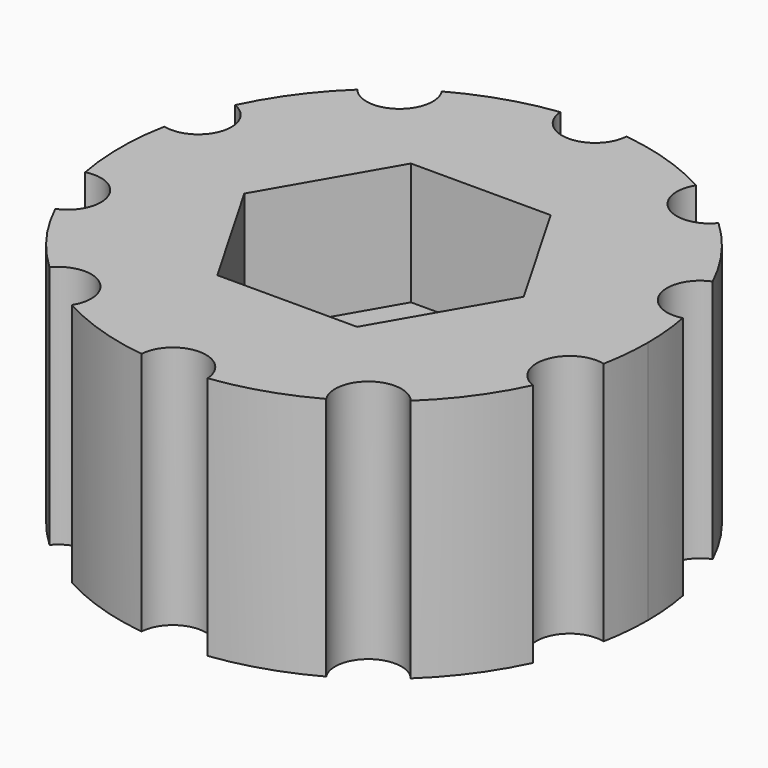
from build123d import *

# Parameters (mm, degrees)
F1_DEPTH = 10
F2_R     = 3
F3_DEPTH = 10.001
F4_R     = 3
F5_DEPTH = 5


with BuildPart() as f1:
    # F0 (on Top) → F1 (new body)
    with BuildSketch(Plane.XY):
        with BuildLine():
            ThreePointArc((10.6036903919, -2.023307953), (10.747066176, -1.0161661329), (10.795, 0))
            ThreePointArc((10.795, 0), (10.747066176, 1.0161661329), (10.6036903919, 2.023307953))
            ThreePointArc((10.6036903919, 2.023307953), (8.9778667931, 2.9170857512), (9.7678363058, 4.5958023134))
            ThreePointArc((9.7678363058, 4.5958023134), (8.7333384543, 6.3451417985), (7.3892951545, 7.8695833511))
            ThreePointArc((7.3892951545, 7.8695833511), (5.5486268246, 7.6370296448), (5.2010007473, 9.4594723017))
            ThreePointArc((5.2010007473, 9.4594723017), (3.3358384543, 10.2666550934), (1.352440321, 10.7099453863))
            ThreePointArc((1.352440321, 10.7099453863), (0, 9.4398877872), (-1.352440321, 10.7099453863))
            ThreePointArc((-1.352440321, 10.7099453863), (-3.3358384543, 10.2666550934), (-5.2010007473, 9.4594723017))
            ThreePointArc((-5.2010007473, 9.4594723017), (-5.0438407916, 9.1114188675), (-4.9900295857, 8.7333384543))
            ThreePointArc((-4.9900295857, 8.7333384543), (-5.8861297374, 7.4583337339), (-7.3892951545, 7.8695833511))
            ThreePointArc((-7.3892951545, 7.8695833511), (-8.7333384543, 6.3451417985), (-9.7678363058, 4.5958023134))
            ThreePointArc((-9.7678363058, 4.5958023134), (-9.1458775641, 4.0975384208), (-8.9115428806, 3.3358384543))
            ThreePointArc((-8.9115428806, 3.3358384543), (-9.4361105551, 2.2650794341), (-10.6036903919, 2.023307953))
            ThreePointArc((-10.6036903919, 2.023307953), (-10.795, 0), (-10.6036903919, -2.023307953))
            ThreePointArc((-10.6036903919, -2.023307953), (-9.4361105551, -2.2650794341), (-8.9115428806, -3.3358384543))
            ThreePointArc((-8.9115428806, -3.3358384543), (-9.1458775641, -4.0975384208), (-9.7678363058, -4.5958023134))
            ThreePointArc((-9.7678363058, -4.5958023134), (-8.7333384543, -6.3451417985), (-7.3892951545, -7.8695833511))
            ThreePointArc((-7.3892951545, -7.8695833511), (-5.8861297374, -7.4583337339), (-4.9900295857, -8.7333384543))
            ThreePointArc((-4.9900295857, -8.7333384543), (-5.0438407916, -9.1114188675), (-5.2010007473, -9.4594723017))
            ThreePointArc((-5.2010007473, -9.4594723017), (-3.3358384543, -10.2666550934), (-1.352440321, -10.7099453863))
            ThreePointArc((-1.352440321, -10.7099453863), (0, -9.4398877872), (1.352440321, -10.7099453863))
            ThreePointArc((1.352440321, -10.7099453863), (3.3358384543, -10.2666550934), (5.2010007473, -9.4594723017))
            ThreePointArc((5.2010007473, -9.4594723017), (5.5486268246, -7.6370296448), (7.3892951545, -7.8695833511))
            ThreePointArc((7.3892951545, -7.8695833511), (8.7333384543, -6.3451417985), (9.7678363058, -4.5958023134))
            ThreePointArc((9.7678363058, -4.5958023134), (8.9778667931, -2.9170857512), (10.6036903919, -2.023307953))
        make_face()
    extrude(amount=F1_DEPTH)

    # F2 (on face) → F3 (cut, through all)
    with BuildSketch(Plane.XY.offset(10)):
        Circle(F2_R)
    extrude(amount=-F3_DEPTH, mode=Mode.SUBTRACT)

    # F4 (on face) → F5 (cut)
    with BuildSketch(Plane.XY.offset(10)):
        Polygon((2.8578838325, -4.95), (5.715767665, 0), (2.8578838325, 4.95), (-2.8578838325, 4.95), (-5.715767665, 0), (-2.8578838325, -4.95), align=None)
        Circle(F4_R, mode=Mode.SUBTRACT)
    extrude(amount=-F5_DEPTH, mode=Mode.SUBTRACT)


solid = f1.part
